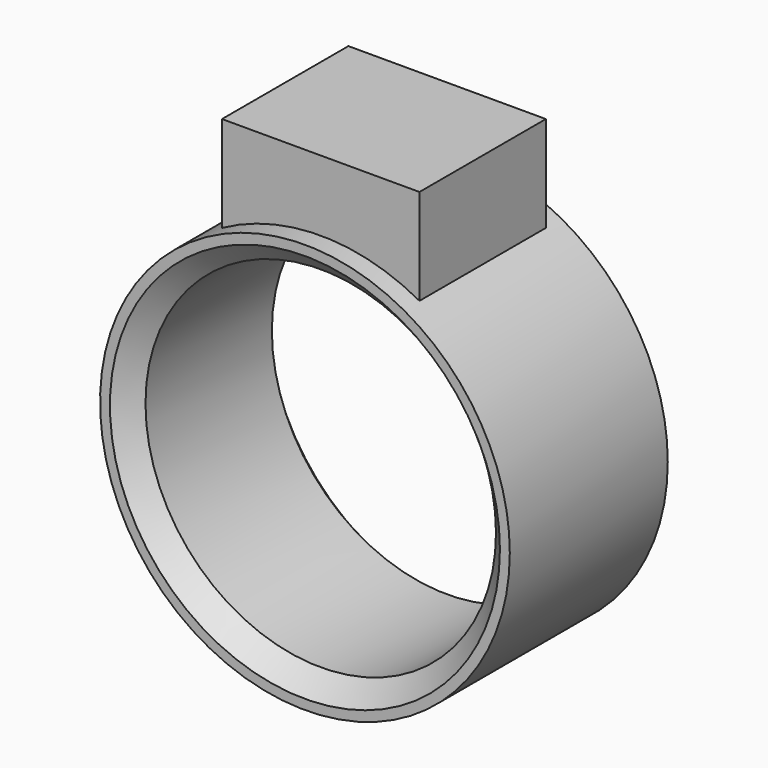
from build123d import *

# Parameters (mm, degrees)
F0_R          = 8.875
F1_DEPTH      = 5
F1_DEPTH_BACK = 5
F2_DEPTH      = 4
F2_DEPTH_BACK = 4
F3_SIZE       = 1


# Not quite as in the source:
# - a feature names something its author has since deleted; it is built from what else it names


with BuildPart() as f1:
    # F0 (on Front) → F1 (new body, two sides)
    with BuildSketch(Plane.XZ) as f1_sk:
        with BuildLine():
            ThreePointArc((-5, 9.0906889178), (-5.2804178338, -8.9307229551), (10.375, 0))
            ThreePointArc((10.375, 0), (8.9307229551, 5.2804178338), (5, 9.0906889178))
            Line((5, 9.0906889178), (5, 8.9453239366))
            Line((5, 8.9453239366), (-5, 8.9453239366))
            Line((-5, 8.9453239366), (-5, 9.0906889178))
        make_face()
        Circle(F0_R, mode=Mode.SUBTRACT)
        with BuildLine():
            Line((5, 8.9453239366), (5, 9.0906889178))
            ThreePointArc((5, 9.0906889178), (0, 10.375), (-5, 9.0906889178))
            Line((-5, 9.0906889178), (-5, 8.9453239366))
            Line((-5, 8.9453239366), (5, 8.9453239366))
        make_face()
    extrude(amount=F1_DEPTH)
    extrude(f1_sk.sketch, amount=-F1_DEPTH_BACK)

    # F0 (on Front) → F2 (join, two sides)
    with BuildSketch(Plane.XZ) as f2_sk:
        with BuildLine():
            ThreePointArc((-5, 9.0906889178), (0, 10.375), (5, 9.0906889178))
            Line((5, 9.0906889178), (5, 13.9453239366))
            Line((5, 13.9453239366), (-5, 13.9453239366))
            Line((-5, 13.9453239366), (-5, 9.0906889178))
        make_face()
    extrude(amount=F2_DEPTH)
    extrude(f2_sk.sketch, amount=-F2_DEPTH_BACK)

    # F3
    f3_edges = [f1.edges().sort_by_distance(p)[0] for p in [
        (-8.875, 5, 0),
        (-8.875, -5, 0),
    ]]
    chamfer(f3_edges, length=F3_SIZE)


solid = f1.part
